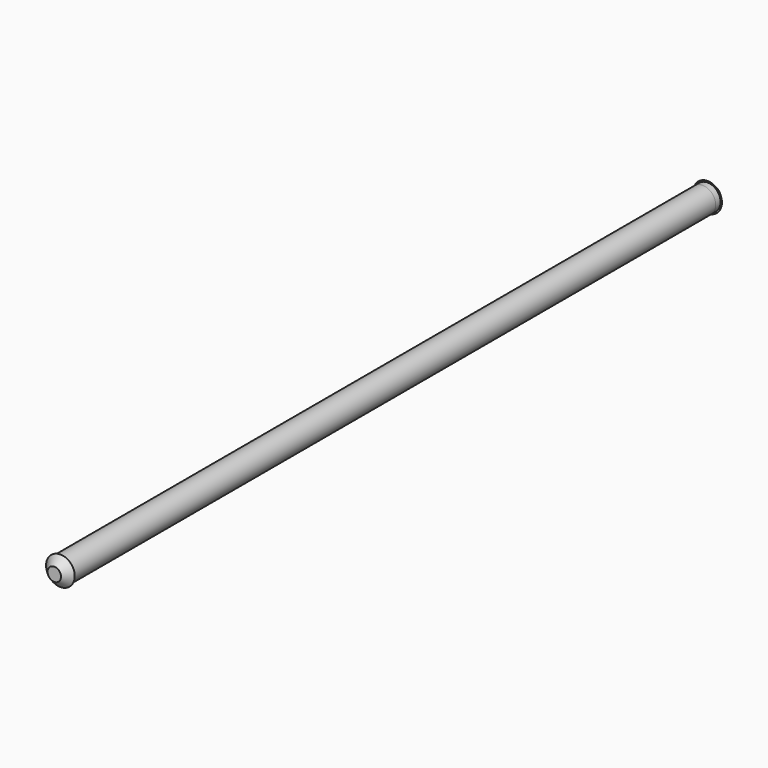
from build123d import *

# Parameters (mm, degrees)
F0_R     = 1.0795
F1_DEPTH = 66.802
F2_R     = 1.0795
F3_DEPTH = 0.508
F4_R     = 1.2446
F4_R_2   = 1.0795
F5_DEPTH = 0.635


# Not quite as in the source:
# - a fillet or chamfer that OpenCascade refuses, or shapes differently, is made with other operations: its cross-section is extruded or revolved along the edge and cut away or added
# - two fillets or chamfers of one size are made in one step
# - a feature of the source that left no trace in its solid (it failed there, or was rolled back) is left out
# - a pattern or mirror of a feature is missing from the dataset's text; its kind, count and spacing are read off the source's solid


with BuildPart() as f1:
    # F0 (on Front) → F1 (new body)
    with BuildSketch(Plane.XZ):
        with Locations((9.3034878373, 10.9315989539)):
            Circle(F0_R)
    extrude(amount=F1_DEPTH)

    # F2 (on face) → F3 (join)
    with BuildSketch(Plane(origin=(0, 0, 0), x_dir=(-1, 0, 0), z_dir=(0, 1, 0))):
        with Locations((-9.3034878373, 10.9315989539)):
            Circle(F2_R)
    extrude(amount=F3_DEPTH)

    # F4 (on face) → F5 (join)
    with BuildSketch(Plane.XZ.offset(66.802)):
        with Locations((9.3034878373, 10.9315989539)):
            Circle(F4_R)
        with Locations((9.3034878373, 10.9315989539)):
            Circle(F4_R_2, mode=Mode.SUBTRACT)
        with Locations((9.3034878373, 10.9315989539)):
            Circle(F4_R_2)
    f5 = extrude(amount=F5_DEPTH)

    # F5_copies: F5 across plane
    add(f5.mirror(Plane.ZX.offset(-33.147)))

    # F8: chamfer of 0.6858 on 2 edges, made by hand

    # F8_s1 → F8_t2 (revolve, cut)
    with BuildSketch(Plane.XY.offset(10.9315989539)):
        Polygon((10.5480878373, 0.4572), (9.8622878373, 1.143), (10.5480878373, 1.143), align=None)
    revolve(axis=Axis((9.3034878373, 1.143, 10.9315989539), (0, -1, 0)), mode=Mode.SUBTRACT)

    # F8_s3 → F8_t4 (revolve, cut)
    with BuildSketch(Plane.XY.offset(10.9315989539)):
        Polygon((10.5480878373, -66.7512), (9.8622878373, -67.437), (10.5480878373, -67.437), align=None)
    revolve(axis=Axis((9.3034878373, -67.437, 10.9315989539), (0, -1, 0)), mode=Mode.SUBTRACT)


solid = f1.part
